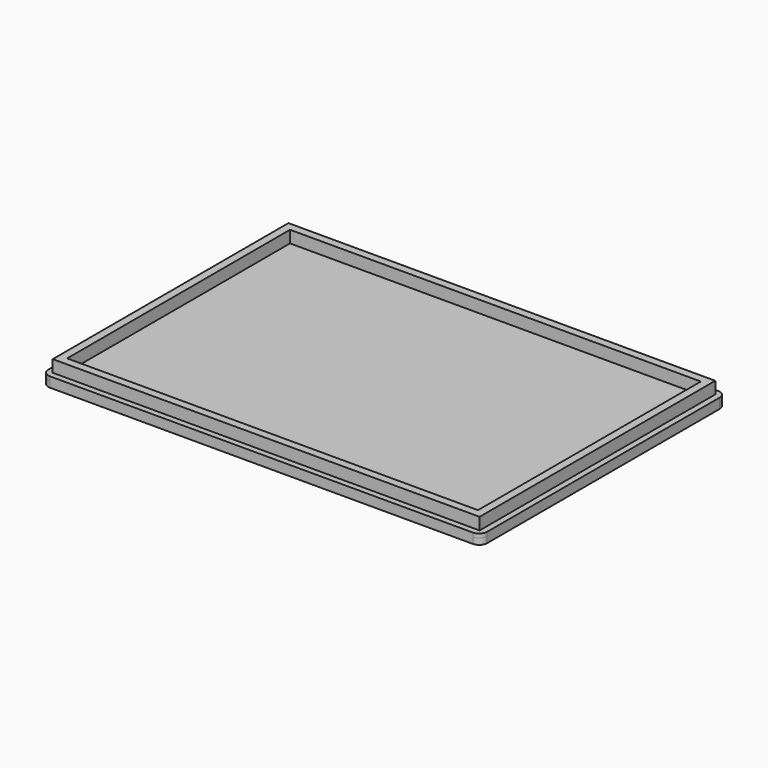
from build123d import *

# Parameters (mm, degrees)
F2_W      = 109.5
F2_H      = 76.5
F3_DEPTH  = 1
F1_W      = 106.5
F1_H      = 73.5
F4_DEPTH  = 3
F0_W      = 102.5
F0_H      = 69.5
F5_DEPTH  = 3
F6_R      = 10.8
F7_DEPTH  = 1
F8_R      = 2.25
F8_R_2    = 1
F9_DEPTH  = 2.5
F10_R     = 7.825
F10_R_2   = 6.575
F11_DEPTH = 0.6
F12_R     = 4.4225
F12_R_2   = 4.4125
F13_DEPTH = 0.6
F14_R     = 0.59999
F15_R     = 2
F16_R     = 15.5
F17_DEPTH = 1.5


# Not quite as in the source:
# - a fillet or chamfer is up to 0.001 mm smaller than in the source, because OpenCascade refuses the exact size


with BuildPart() as f3:
    # F2 (on Top) → F3 (new body)
    with BuildSketch(Plane.XY):
        Rectangle(F2_W, F2_H)
    extrude(amount=-F3_DEPTH)

    # F1 (on Top) → F4 (join)
    with BuildSketch(Plane.XY):
        Rectangle(F1_W, F1_H)
    extrude(amount=F4_DEPTH)

    # F0 (on Top) → F5 (cut, through all)
    with BuildSketch(Plane.XY):
        Rectangle(F0_W, F0_H)
    extrude(amount=F5_DEPTH, mode=Mode.SUBTRACT)

    # F6 (on face) → F7 (join)
    with BuildSketch(Plane(origin=(0, 0, -1), x_dir=(1, 0, 0), z_dir=(0, 0, -1))):
        Circle(F6_R)
    extrude(amount=F7_DEPTH)

    # F8 (on face) → F9 (join)
    with BuildSketch(Plane(origin=(0, 0, -1), x_dir=(1, 0, 0), z_dir=(0, 0, -1))):
        Circle(F8_R)
        Circle(F8_R_2, mode=Mode.SUBTRACT)
    extrude(amount=F9_DEPTH)

    # F10 (on face) → F11 (join)
    with BuildSketch(Plane(origin=(0, 0, -2), x_dir=(1, 0, 0), z_dir=(0, 0, -1))):
        Circle(F10_R)
        Circle(F10_R_2, mode=Mode.SUBTRACT)
    extrude(amount=F11_DEPTH)

    # F12 (on face) → F13 (join)
    with BuildSketch(Plane(origin=(0, 0, -2), x_dir=(1, 0, 0), z_dir=(0, 0, -1))):
        Circle(F12_R)
        Circle(F12_R_2, mode=Mode.SUBTRACT)
    extrude(amount=F13_DEPTH)

    # F14 (radius 0.6 in the source; OpenCascade refuses exactly that, so slightly less here)
    f14_edges = [f3.edges().sort_by_distance(p)[0] for p in [
        (-4.4225, 0, -2),
        (-6.575, 0, -2),
        (-2.25, 0, -2),
        (-4.4125, 0, -2),
    ]]
    fillet(f14_edges, radius=F14_R)

    # F15
    f15_edges = [f3.edges().sort_by_distance(p)[0] for p in [
        (-54.75, -38.25, -0.5),
        (54.75, -38.25, -0.5),
        (54.75, 38.25, -0.5),
        (-54.75, 38.25, -0.5),
    ]]
    fillet(f15_edges, radius=F15_R)

    # F16 (on face) → F17 (join)
    with BuildSketch(Plane(origin=(0, 0, -1), x_dir=(1, 0, 0), z_dir=(0, 0, -1))):
        with BuildLine():
            ThreePointArc((-52.75, 38.25), (-54.1642135624, 37.6642135624), (-54.75, 36.25))
            Line((-54.75, 36.25), (-54.75, -36.25))
            ThreePointArc((-54.75, -36.25), (-54.1642135624, -37.6642135624), (-52.75, -38.25))
            Line((-52.75, -38.25), (52.75, -38.25))
            ThreePointArc((52.75, -38.25), (54.1642135624, -37.6642135624), (54.75, -36.25))
            Line((54.75, -36.25), (54.75, 36.25))
            ThreePointArc((54.75, 36.25), (54.1642135624, 37.6642135624), (52.75, 38.25))
            Line((52.75, 38.25), (-52.75, 38.25))
        make_face()
        Circle(F16_R, mode=Mode.SUBTRACT)
    extrude(amount=F17_DEPTH)


solid = f3.part
